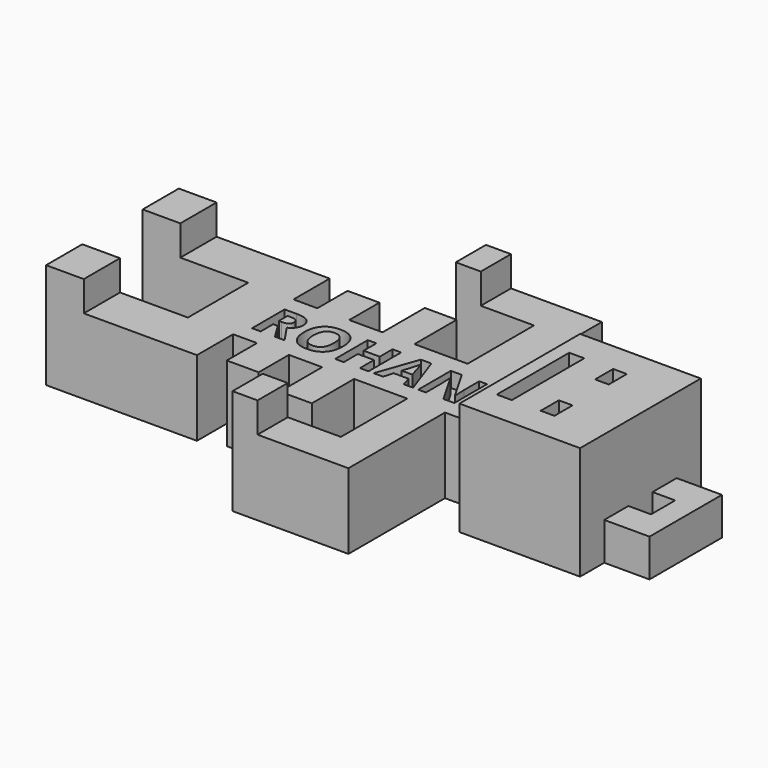
from build123d import *

# Parameters (mm, degrees)
F0_W         = 20.32
F0_H         = 25.4
F1_DEPTH     = 19.05
F2_W         = 6.6547346413
F2_H         = 7.62
F2_W_2       = 5.3730774671
F2_H_2       = 6.35
F2_H_3       = 12.7
F2_W_3       = 5.6027897402
F2_H_4       = 8.89
F2_W_4       = 8.952341345
F2_W_5       = 6.35
F2_H_5       = 13.97
F2_W_6       = 7.5133969746
F2_W_7       = 13.1662150379
F3_DEPTH     = 12.7
F4_TEXT_SIZE = 9.6128405491
F5_DEPTH     = 2.54
F6_W         = 6.35
F6_H         = 7.62
F6_W_2       = 4.2138736929
F6_H_2       = 6.35
F7_DEPTH     = 5.08
F8_W         = 2.54
F8_H         = 15.24
F8_W_2       = 2.3044385016
F8_H_2       = 3.81
F9_DEPTH     = 2.54
F10_W        = 15.24
F10_H        = 6.35
F11_DEPTH    = 7.62
F12_DEPTH    = 2.54


# Not quite as in the source:
# - Text() gives the source's letters only with a copy of the font that has no kerning and outlines rounded to 1/6400 em; it was checked with that copy


with BuildPart() as f1:
    # F0 (on Top) → F1 (new body)
    with BuildSketch(Plane.XY):
        with Locations((33.8114820788, 0)):
            Rectangle(F0_W, F0_H)
    extrude(amount=F1_DEPTH)

    # F2 (on Top) → F3 (join)
    with BuildSketch(Plane.XY):
        Polygon((-38.2737832799, 6.35), (-27.1485179212, 6.35), (-27.1485179212, -6.35), (-38.2737832799, -6.35), (-38.2737832799, -13.97), (-19.5285179212, -13.97), (-19.5285179212, -6.35), (-15.5132009152, -6.35), (-15.5132009152, 6.35), (-19.5285179212, 6.35), (-19.5285179212, 13.97), (-38.2737832799, 13.97), align=None)
        with Locations((-41.6011506005, 10.16)):
            Rectangle(F2_W, F2_H)
        with Locations((-41.6011506005, -10.16)):
            Rectangle(F2_W, F2_H)
        with Locations((-12.8266621816, 9.525)):
            Rectangle(F2_W_2, F2_H_2)
        with Locations((-12.8266621816, 0)):
            Rectangle(F2_W_2, F2_H_3)
        with Locations((-12.8266621816, -9.525)):
            Rectangle(F2_W_2, F2_H_2)
        with Locations((-7.338728578, 0)):
            Rectangle(F2_W_3, F2_H_3)
        with Locations((-1.8507949743, 10.795)):
            Rectangle(F2_W_2, F2_H_4)
        with Locations((-1.8507949743, 0)):
            Rectangle(F2_W_2, F2_H_3)
        with Locations((-1.8507949743, -10.795)):
            Rectangle(F2_W_2, F2_H_4)
        with Locations((5.3119144317, 0)):
            Rectangle(F2_W_4, F2_H_3)
        with Locations((12.9630851042, 13.335)):
            Rectangle(F2_W_5, F2_H_5)
        with Locations((12.9630851042, 0)):
            Rectangle(F2_W_5, F2_H_3)
        with Locations((12.9630851042, -13.335)):
            Rectangle(F2_W_5, F2_H_5)
        with Locations((19.8947835915, 0)):
            Rectangle(F2_W_6, F2_H_3)
        with Locations((3.2049775852, 23.495)):
            Rectangle(F2_W_7, F2_H_2)
        with Locations((12.9630851042, 23.495)):
            Rectangle(F2_W_5, F2_H_2)
        with Locations((12.9630851042, -23.495)):
            Rectangle(F2_W_5, F2_H_2)
        with Locations((3.2049775852, -23.495)):
            Rectangle(F2_W_7, F2_H_2)
        Polygon((51.5914820788, 7.62), (43.9714820788, 7.62), (43.9714820788, 2.54), (47.7814820788, 2.54), (47.7814820788, -2.54), (43.9714820788, -2.54), (43.9714820788, -7.62), (51.5914820788, -7.62), align=None)
    extrude(amount=F3_DEPTH)

    # F4 (on face) → F5 (cut)
    with BuildSketch(Plane.XY.offset(12.7)):
        with Locations((-19.5285179212, -3.4606225977)):
            Text('ROHAN', F4_TEXT_SIZE, font='Open Sans', font_style=FontStyle.BOLD, text_align=(TextAlign.LEFT, TextAlign.BOTTOM))
    extrude(amount=-F5_DEPTH, mode=Mode.SUBTRACT)

    # F6 (on face) → F7 (join)
    with BuildSketch(Plane.XY.offset(12.7)):
        with Locations((-41.7535179212, 10.16)):
            Rectangle(F6_W, F6_H)
        with Locations((-41.7535179212, -10.16)):
            Rectangle(F6_W, F6_H)
        with Locations((-1.2711930872, 23.495)):
            Rectangle(F6_W_2, F6_H_2)
        with Locations((-1.2711930872, -23.495)):
            Rectangle(F6_W_2, F6_H_2)
    extrude(amount=F7_DEPTH)

    # F8 (on face) → F9 (cut)
    with BuildSketch(Plane.XY.offset(19.05)):
        with Locations((27.1470436171, 0)):
            Rectangle(F8_W, F8_H)
        with Locations((34.4282668084, 5.715)):
            Rectangle(F8_W_2, F8_H_2)
        with Locations((34.4282668084, -5.715)):
            Rectangle(F8_W_2, F8_H_2)
    extrude(amount=-F9_DEPTH, mode=Mode.SUBTRACT)

    # F10 (on face) → F11 (cut, through all)
    with BuildSketch(Plane.YZ.offset(51.5914820788)):
        with Locations((0, 9.525)):
            Rectangle(F10_W, F10_H)
    extrude(amount=-F11_DEPTH, mode=Mode.SUBTRACT)

    # F4 (on face) → F12 (cut)
    with BuildSketch(Plane.XY.offset(12.7)):
        with Locations((-19.5285179212, -3.4606225977)):
            Text('ROHAN', F4_TEXT_SIZE, font='Open Sans', font_style=FontStyle.BOLD, text_align=(TextAlign.LEFT, TextAlign.BOTTOM))
    extrude(amount=F12_DEPTH, mode=Mode.SUBTRACT)


solid = f1.part
